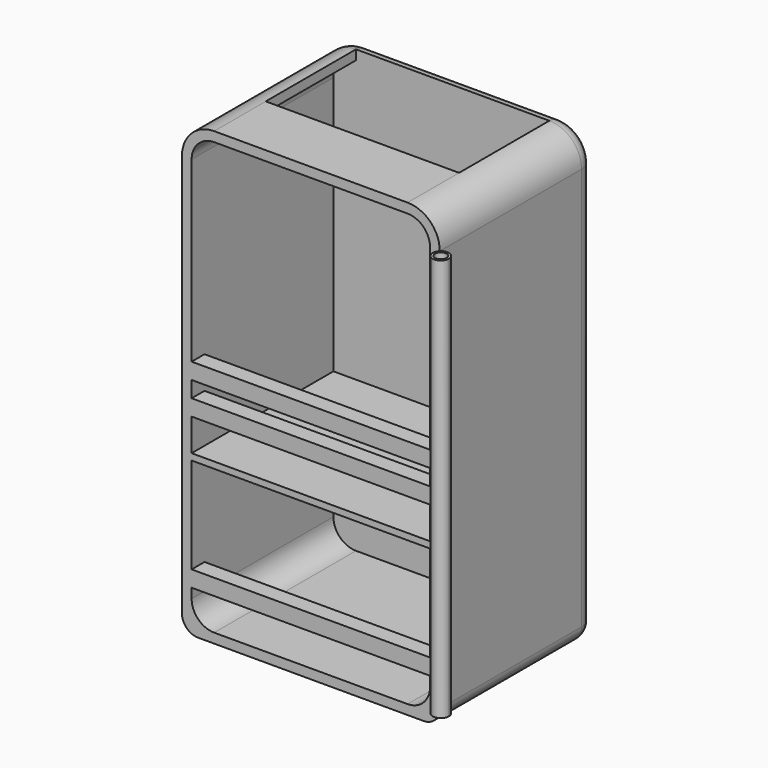
from build123d import *

# Parameters (mm, degrees)
F0_W      = 80
F0_H      = 60
F1_DEPTH  = 140
F2_R      = 10
F3_R      = 10
F4_R      = 5
F5_R      = 5
F7_DEPTH  = 55
F9_W      = 74
F9_H      = 2
F10_DEPTH = 55
F11_W     = 60
F11_H     = 35
F12_DEPTH = 28
F13_R     = 4.99999
F14_W     = 5
F14_H     = 5
F15_DEPTH = 74
F16_W     = 5
F16_H     = 5
F17_DEPTH = 74
F18_R     = 2.5
F19_DEPTH = 130
F20_DEPTH = 5
F21_W     = 5
F21_H     = 5
F22_DEPTH = 74
F23_R     = 1.8
F24_DEPTH = 132


# Not quite as in the source:
# - a fillet or chamfer is up to 0.001 mm smaller than in the source, because OpenCascade refuses the exact size
# - a feature names something its author has since deleted; it is built from what else it names


with BuildPart() as f1:
    # F0 (on Top) → F1 (new body)
    with BuildSketch(Plane.XY):
        with Locations((-5.2340733026, -14.0806569159)):
            Rectangle(F0_W, F0_H)
    extrude(amount=F1_DEPTH)

    # F2
    f2_edges = [f1.edges().sort_by_distance(p)[0] for p in [
        (-45.234073, -14.080657, 140),
    ]]
    fillet(f2_edges, radius=F2_R)

    # F3
    f3_edges = [f1.edges().sort_by_distance(p)[0] for p in [
        (34.765927, -14.080657, 140),
    ]]
    fillet(f3_edges, radius=F3_R)

    # F4
    f4_edges = [f1.edges().sort_by_distance(p)[0] for p in [
        (-45.234073, -14.080657, 0),
    ]]
    fillet(f4_edges, radius=F4_R)

    # F5
    f5_edges = [f1.edges().sort_by_distance(p)[0] for p in [
        (34.765927, -14.080657, 0),
    ]]
    fillet(f5_edges, radius=F5_R)

    # F6 (on face) → F7 (cut)
    with BuildSketch(Plane.XZ.offset(44.0806569159)):
        with BuildLine():
            Line((24.7659266974, 137), (-35.2340733026, 137))
            ThreePointArc((-35.2340733026, 137), (-40.1838207709, 134.9497474683), (-42.2340733026, 130))
            Line((-42.2340733026, 130), (-42.2340733026, 10))
            ThreePointArc((-42.2340733026, 10), (-40.1838207709, 5.0502525317), (-35.2340733026, 3))
            Line((-35.2340733026, 3), (24.7659266974, 3))
            ThreePointArc((24.7659266974, 3), (29.7156741658, 5.0502525317), (31.7659266974, 10))
            Line((31.7659266974, 10), (31.7659266974, 130))
            ThreePointArc((31.7659266974, 130), (29.7156741658, 134.9497474683), (24.7659266974, 137))
        make_face()
    extrude(amount=-F7_DEPTH, mode=Mode.SUBTRACT)

    # F9 (on face) → F10 (join)
    with BuildSketch(Plane.XZ.offset(-10.9193430841)):
        with Locations((-5.2340733026, 48.7519614398)):
            Rectangle(F9_W, F9_H)
    extrude(amount=F10_DEPTH)

    # F11 (on face) → F12 (cut)
    with BuildSketch(Plane.XY.offset(140)):
        with Locations((-5.2340733026, -6.5806569159)):
            Rectangle(F11_W, F11_H)
    extrude(amount=-F12_DEPTH, mode=Mode.SUBTRACT)

    # F13 (radius 5 in the source; OpenCascade refuses exactly that, so slightly less here)
    f13_edges = [f1.edges().sort_by_distance(p)[0] for p in [
        (-5.234073, 15.919343, 140),
    ]]
    fillet(f13_edges, radius=F13_R)

    # F14 (on face) → F15 (join)
    with BuildSketch(Plane.YZ.offset(-42.2340733026)):
        with Locations((-41.5806569159, 62.2519614398)):
            Rectangle(F14_W, F14_H)
    extrude(amount=F15_DEPTH)

    # F16 (on face) → F17 (join)
    with BuildSketch(Plane.YZ.offset(-42.2340733026)):
        with Locations((-41.5806569159, 72.2519614398)):
            Rectangle(F16_W, F16_H)
    extrude(amount=F17_DEPTH)

    # F18 (on Top) → F19 (join)
    with BuildSketch(Plane.XY):
        with Locations((36.524810933, -45.8572621748)):
            Circle(F18_R)
    extrude(amount=F19_DEPTH)

    # F20 (cut): a face of the model
    f20_faces = [f1.faces().sort_by_distance(p)[0] for p in [
        (36.524810933, -45.8572621748, 0),
    ]]
    extrude(f20_faces, amount=-F20_DEPTH, mode=Mode.SUBTRACT)

    # F21 (on face) → F22 (join)
    with BuildSketch(Plane.YZ.offset(-42.2340733026)):
        with Locations((-41.5806569159, 15.5)):
            Rectangle(F21_W, F21_H)
    extrude(amount=F22_DEPTH)

    # F23 (on face) → F24 (cut)
    with BuildSketch(Plane.XY.offset(130)):
        with Locations((36.524810933, -45.8572621748)):
            Circle(F23_R)
    extrude(amount=-F24_DEPTH, mode=Mode.SUBTRACT)


solid = f1.part
